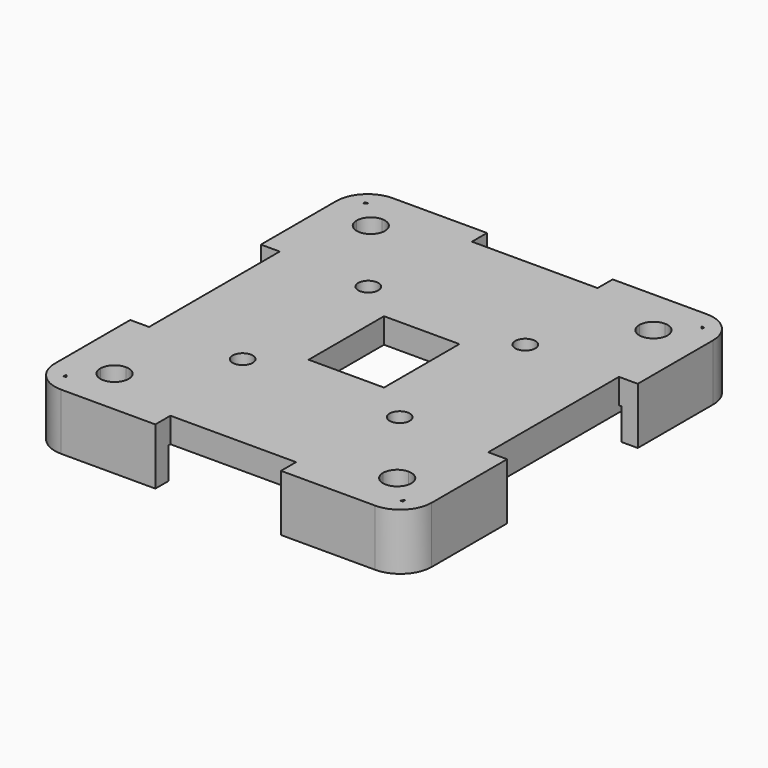
from build123d import *

# Parameters (mm, degrees)
F0_R     = 1.6
F0_W     = 12
F0_H     = 15
F1_DEPTH = 4
F2_R     = 2.25
F3_DEPTH = 1
F4_DEPTH = 5
F5_R     = 5


# Not quite as in the source:
# - ends of sketch curves that miss each other by under 0.0002 mm in the source are joined


with BuildPart() as f1:
    # F0 (on Top) → F1 (new body)
    with BuildSketch(Plane.XY):
        Polygon((-26.600003, -29.899997), (-26.5, -30), (-10, -30), (10, -30), (26.5, -30), (26.6, -29.9), (27, -29.5), (27, -13), (27, 13), (27, 29.5), (26.5999975, 29.9000025), (26.5, 30), (10, 30), (-10, 30), (-26.5, 30), (-26.599999, 29.900001), (-27, 29.5), (-27, 13), (-27, -13), (-27, -29.5), align=None)
        with BuildLine():
            ThreePointArc((-22.5, -23.25), (-20.9090097423, -23.9090097423), (-20.25, -25.5))
            ThreePointArc((-20.25, -25.5), (-20.9090097423, -27.0909902577), (-22.5, -27.75))
            ThreePointArc((-22.5, -27.75), (-24.0909902577, -27.0909902577), (-24.75, -25.5))
            ThreePointArc((-24.75, -25.5), (-24.0909902577, -23.9090097423), (-22.5, -23.25))
        make_face(mode=Mode.SUBTRACT)
        with Locations((-12.5, -12.5)):
            Circle(F0_R, mode=Mode.SUBTRACT)
        with BuildLine():
            ThreePointArc((22.5, -23.25), (24.0909902577, -23.9090097423), (24.75, -25.5))
            ThreePointArc((24.75, -25.5), (24.0909902577, -27.0909902577), (22.5, -27.75))
            ThreePointArc((22.5, -27.75), (20.9090097423, -27.0909902577), (20.25, -25.5))
            ThreePointArc((20.25, -25.5), (20.9090097423, -23.9090097423), (22.5, -23.25))
        make_face(mode=Mode.SUBTRACT)
        with Locations((12.5, -12.5)):
            Circle(F0_R, mode=Mode.SUBTRACT)
        with Locations((-12.5, 12.5)):
            Circle(F0_R, mode=Mode.SUBTRACT)
        with BuildLine():
            ThreePointArc((-22.5, 27.75), (-20.9090097423, 27.0909902577), (-20.25, 25.5))
            ThreePointArc((-20.25, 25.5), (-20.9090097423, 23.9090097423), (-22.5, 23.25))
            ThreePointArc((-22.5, 23.25), (-24.0909902577, 23.9090097423), (-24.75, 25.5))
            ThreePointArc((-24.75, 25.5), (-24.0909902577, 27.0909902577), (-22.5, 27.75))
        make_face(mode=Mode.SUBTRACT)
        Rectangle(F0_W, F0_H, mode=Mode.SUBTRACT)
        with Locations((12.5, 12.5)):
            Circle(F0_R, mode=Mode.SUBTRACT)
        with BuildLine():
            ThreePointArc((22.5, 27.75), (24.0909902577, 27.0909902577), (24.75, 25.5))
            ThreePointArc((24.75, 25.5), (24.0909902577, 23.9090097423), (22.5, 23.25))
            ThreePointArc((22.5, 23.25), (20.9090097423, 23.9090097423), (20.25, 25.5))
            ThreePointArc((20.25, 25.5), (20.9090097423, 27.0909902577), (22.5, 27.75))
        make_face(mode=Mode.SUBTRACT)
        Polygon((-10, -30), (-26.5, -30), (-26.6, -30), (-27, -30), (-27, -29.5), (-27, -13), (-30, -13), (-30, -33), (-10, -33), align=None)
        Polygon((26.5, -30), (10, -30), (10, -33), (30, -33), (30, -13), (27, -13), (27, -29.5), (27, -30), (26.6, -30), align=None)
        Polygon((27, 29.5), (27, 13), (30, 13), (30, 33), (10, 33), (10, 30), (26.5, 30), (26.6, 30), (27, 30), align=None)
        Polygon((-30, 13), (-27, 13), (-27, 29.5), (-27, 30), (-26.6, 30), (-26.5, 30), (-10, 30), (-10, 33), (-30, 33), align=None)
    extrude(amount=F1_DEPTH)

    # F2 (on face) → F3 (join)
    with BuildSketch(Plane(origin=(0, 0, 0), x_dir=(1, 0, 0), z_dir=(0, 0, -1))):
        Polygon((-16.5, -30), (-16.5, 30), (-26.5, 30), (-27, 29.5), (-27, 13), (-27, -13), (-27, -29.500004), (-26.5, -30), align=None)
        with Locations((-22.5, -25.5)):
            Circle(F2_R, mode=Mode.SUBTRACT)
        with Locations((-22.5, 25.5)):
            Circle(F2_R, mode=Mode.SUBTRACT)
        Polygon((27, -13), (27, 13), (27, 29.5), (26.5, 30), (16.5, 30), (16.5, -30), (26.5, -30), (27, -29.500004), align=None)
        with Locations((22.5, -25.5)):
            Circle(F2_R, mode=Mode.SUBTRACT)
        with Locations((22.5, 25.5)):
            Circle(F2_R, mode=Mode.SUBTRACT)
    extrude(amount=F3_DEPTH)

    # F2 (on face) + F0 (on Top) → F4 (join)
    with BuildSketch(Plane(origin=(0, 0, 0), x_dir=(1, 0, 0), z_dir=(0, 0, -1))):
        Polygon((-30, 13), (-27.4, 13), (-27.4, 30.4), (-10, 30.4), (-10, 33), (-30, 33), align=None)
        Polygon((-27.4, -30.4), (-27.4, -13), (-30, -13), (-30, -33), (-10, -33), (-10, -30.4), align=None)
        Polygon((27.4, -30.4), (10, -30.4), (10, -33), (30, -33), (30, -13), (27.4, -13), align=None)
    with BuildSketch(Plane.XY):
        Polygon((26.5, -30), (10, -30), (10, -33), (30, -33), (30, -13), (27, -13), (27, -29.5), (27, -30), (26.6, -30), align=None)
    extrude(amount=F4_DEPTH, dir=(0, 0, -1))

    # F5
    f5_edges = [f1.edges().sort_by_distance(p)[0] for p in [
        (30, -33, -0.5),
        (30, 33, -0.5),
        (-30, 33, -0.5),
        (-30, -33, -0.5),
    ]]
    fillet(f5_edges, radius=F5_R)


solid = f1.part
